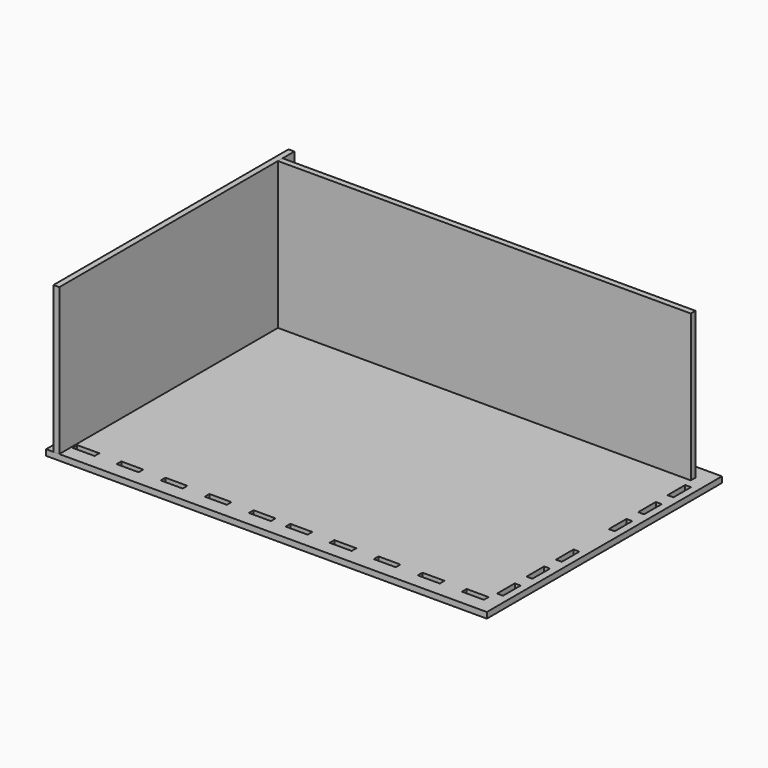
from build123d import *

# Parameters (mm, degrees)
F1_W      = 300
F1_H      = 200
F1_W_2    = 15
F1_H_2    = 4
F1_W_3    = 4
F1_H_3    = 15
F2_DEPTH  = 4
F3_W      = 4
F3_H      = 15
F4_DEPTH  = 4
F5_W      = 4
F5_H      = 200
F6_DEPTH  = 100
F8_W      = 15
F8_H      = 4
F9_DEPTH  = 4
F10_W     = 281
F10_H     = 4
F11_DEPTH = 100


with BuildPart() as f2:
    # F1 (on Top) → F2 (new body)
    with BuildSketch(Plane.XY):
        Rectangle(F1_W, F1_H)
        with Locations((-132.5, -88)):
            Rectangle(F1_W_2, F1_H_2, mode=Mode.SUBTRACT)
        with Locations((-102.5, -88)):
            Rectangle(F1_W_2, F1_H_2, mode=Mode.SUBTRACT)
        with Locations((-143, -72.5)):
            Rectangle(F1_W_3, F1_H_3, mode=Mode.SUBTRACT)
        with Locations((-72.5, -88)):
            Rectangle(F1_W_2, F1_H_2, mode=Mode.SUBTRACT)
        with Locations((-42.5, -88)):
            Rectangle(F1_W_2, F1_H_2, mode=Mode.SUBTRACT)
        with Locations((-12.5, -88)):
            Rectangle(F1_W_2, F1_H_2, mode=Mode.SUBTRACT)
        with Locations((-143, -47.5)):
            Rectangle(F1_W_3, F1_H_3, mode=Mode.SUBTRACT)
        with Locations((-143, -22.5)):
            Rectangle(F1_W_3, F1_H_3, mode=Mode.SUBTRACT)
        with Locations((12.5, -88)):
            Rectangle(F1_W_2, F1_H_2, mode=Mode.SUBTRACT)
        with Locations((42.5, -88)):
            Rectangle(F1_W_2, F1_H_2, mode=Mode.SUBTRACT)
        with Locations((72.5, -88)):
            Rectangle(F1_W_2, F1_H_2, mode=Mode.SUBTRACT)
        with Locations((102.5, -88)):
            Rectangle(F1_W_2, F1_H_2, mode=Mode.SUBTRACT)
        with Locations((132.5, -88)):
            Rectangle(F1_W_2, F1_H_2, mode=Mode.SUBTRACT)
        with Locations((143, -72.5)):
            Rectangle(F1_W_3, F1_H_3, mode=Mode.SUBTRACT)
        with Locations((143, -47.5)):
            Rectangle(F1_W_3, F1_H_3, mode=Mode.SUBTRACT)
        with Locations((143, -22.5)):
            Rectangle(F1_W_3, F1_H_3, mode=Mode.SUBTRACT)
        with Locations((-143, 22.5)):
            Rectangle(F1_W_3, F1_H_3, mode=Mode.SUBTRACT)
        with Locations((-143, 47.5)):
            Rectangle(F1_W_3, F1_H_3, mode=Mode.SUBTRACT)
        with Locations((-143, 72.5)):
            Rectangle(F1_W_3, F1_H_3, mode=Mode.SUBTRACT)
        with Locations((-132.5, 88)):
            Rectangle(F1_W_2, F1_H_2, mode=Mode.SUBTRACT)
        with Locations((-102.5, 88)):
            Rectangle(F1_W_2, F1_H_2, mode=Mode.SUBTRACT)
        with Locations((-72.5, 88)):
            Rectangle(F1_W_2, F1_H_2, mode=Mode.SUBTRACT)
        with Locations((-42.5, 88)):
            Rectangle(F1_W_2, F1_H_2, mode=Mode.SUBTRACT)
        with Locations((-12.5, 88)):
            Rectangle(F1_W_2, F1_H_2, mode=Mode.SUBTRACT)
        with Locations((143, 22.5)):
            Rectangle(F1_W_3, F1_H_3, mode=Mode.SUBTRACT)
        with Locations((143, 47.5)):
            Rectangle(F1_W_3, F1_H_3, mode=Mode.SUBTRACT)
        with Locations((12.5, 88)):
            Rectangle(F1_W_2, F1_H_2, mode=Mode.SUBTRACT)
        with Locations((42.5, 88)):
            Rectangle(F1_W_2, F1_H_2, mode=Mode.SUBTRACT)
        with Locations((72.5, 88)):
            Rectangle(F1_W_2, F1_H_2, mode=Mode.SUBTRACT)
        with Locations((143, 72.5)):
            Rectangle(F1_W_3, F1_H_3, mode=Mode.SUBTRACT)
        with Locations((102.5, 88)):
            Rectangle(F1_W_2, F1_H_2, mode=Mode.SUBTRACT)
        with Locations((132.5, 88)):
            Rectangle(F1_W_2, F1_H_2, mode=Mode.SUBTRACT)
    extrude(amount=F2_DEPTH)


with BuildPart() as f4:
    # F3 (on face) → F4 (new body)
    with BuildSketch(Plane.XY.offset(4)):
        with Locations((-143, -72.5)):
            Rectangle(F3_W, F3_H)
    extrude(amount=-F4_DEPTH)



with BuildPart() as f4b:
    # F3 (on face) → F4, piece 2 (new body)
    with BuildSketch(Plane.XY.offset(4)):
        with Locations((-143, -47.5)):
            Rectangle(F3_W, F3_H)
    extrude(amount=-F4_DEPTH)


with BuildPart() as f4c:
    # F3 (on face) → F4, piece 3 (new body)
    with BuildSketch(Plane.XY.offset(4)):
        with Locations((-143, -22.5)):
            Rectangle(F3_W, F3_H)
    extrude(amount=-F4_DEPTH)


with BuildPart() as f4d:
    # F3 (on face) → F4, piece 4 (new body)
    with BuildSketch(Plane.XY.offset(4)):
        with Locations((-143, 22.5)):
            Rectangle(F3_W, F3_H)
    extrude(amount=-F4_DEPTH)


with BuildPart() as f4e:
    # F3 (on face) → F4, piece 5 (new body)
    with BuildSketch(Plane.XY.offset(4)):
        with Locations((-143, 47.5)):
            Rectangle(F3_W, F3_H)
    extrude(amount=-F4_DEPTH)


with BuildPart() as f4f:
    # F3 (on face) → F4, piece 6 (new body)
    with BuildSketch(Plane.XY.offset(4)):
        with Locations((-143, 72.5)):
            Rectangle(F3_W, F3_H)
    extrude(amount=-F4_DEPTH)


with BuildPart() as f4_1:
    add(f4.part)

    add(f4b.part)  # F6 merges F4b

    add(f4c.part)  # F6 merges F4c

    add(f4d.part)  # F6 merges F4d

    add(f4e.part)  # F6 merges F4e

    add(f4f.part)  # F6 merges F4f
    # F5 (on face) → F6 (join)
    with BuildSketch(Plane.XY.offset(4)):
        with Locations((-143, 0)):
            Rectangle(F5_W, F5_H)
    extrude(amount=F6_DEPTH)

    # F7: union 


with BuildPart() as f9:
    # F8 (on face) → F9 (new body)
    with BuildSketch(Plane.XY.offset(4)):
        with Locations((-132.5, 88)):
            Rectangle(F8_W, F8_H)
    extrude(amount=-F9_DEPTH)



with BuildPart() as f9b:
    # F8 (on face) → F9, piece 2 (new body)
    with BuildSketch(Plane.XY.offset(4)):
        with Locations((-102.5, 88)):
            Rectangle(F8_W, F8_H)
    extrude(amount=-F9_DEPTH)


with BuildPart() as f9c:
    # F8 (on face) → F9, piece 3 (new body)
    with BuildSketch(Plane.XY.offset(4)):
        with Locations((-72.5, 88)):
            Rectangle(F8_W, F8_H)
    extrude(amount=-F9_DEPTH)


with BuildPart() as f9d:
    # F8 (on face) → F9, piece 4 (new body)
    with BuildSketch(Plane.XY.offset(4)):
        with Locations((-42.5, 88)):
            Rectangle(F8_W, F8_H)
    extrude(amount=-F9_DEPTH)


with BuildPart() as f9e:
    # F8 (on face) → F9, piece 5 (new body)
    with BuildSketch(Plane.XY.offset(4)):
        with Locations((-12.5, 88)):
            Rectangle(F8_W, F8_H)
    extrude(amount=-F9_DEPTH)


with BuildPart() as f9f:
    # F8 (on face) → F9, piece 6 (new body)
    with BuildSketch(Plane.XY.offset(4)):
        with Locations((12.5, 88)):
            Rectangle(F8_W, F8_H)
    extrude(amount=-F9_DEPTH)


with BuildPart() as f9g:
    # F8 (on face) → F9, piece 7 (new body)
    with BuildSketch(Plane.XY.offset(4)):
        with Locations((42.5, 88)):
            Rectangle(F8_W, F8_H)
    extrude(amount=-F9_DEPTH)


with BuildPart() as f9h:
    # F8 (on face) → F9, piece 8 (new body)
    with BuildSketch(Plane.XY.offset(4)):
        with Locations((72.5, 88)):
            Rectangle(F8_W, F8_H)
    extrude(amount=-F9_DEPTH)


with BuildPart() as f9i:
    # F8 (on face) → F9, piece 9 (new body)
    with BuildSketch(Plane.XY.offset(4)):
        with Locations((102.5, 88)):
            Rectangle(F8_W, F8_H)
    extrude(amount=-F9_DEPTH)


with BuildPart() as f9j:
    # F8 (on face) → F9, piece 10 (new body)
    with BuildSketch(Plane.XY.offset(4)):
        with Locations((132.5, 88)):
            Rectangle(F8_W, F8_H)
    extrude(amount=-F9_DEPTH)


with BuildPart() as f9_1:
    add(f9.part)

    add(f9b.part)  # F11 merges F9b

    add(f9c.part)  # F11 merges F9c

    add(f9d.part)  # F11 merges F9d

    add(f9e.part)  # F11 merges F9e

    add(f9f.part)  # F11 merges F9f

    add(f9g.part)  # F11 merges F9g

    add(f9h.part)  # F11 merges F9h

    add(f9i.part)  # F11 merges F9i

    add(f9j.part)  # F11 merges F9j
    # F10 (on face) → F11 (join)
    with BuildSketch(Plane.XY.offset(4)):
        with Locations((-0.5, 88)):
            Rectangle(F10_W, F10_H)
    extrude(amount=F11_DEPTH)


solid = Compound([f2.part, f4_1.part, f9_1.part])
